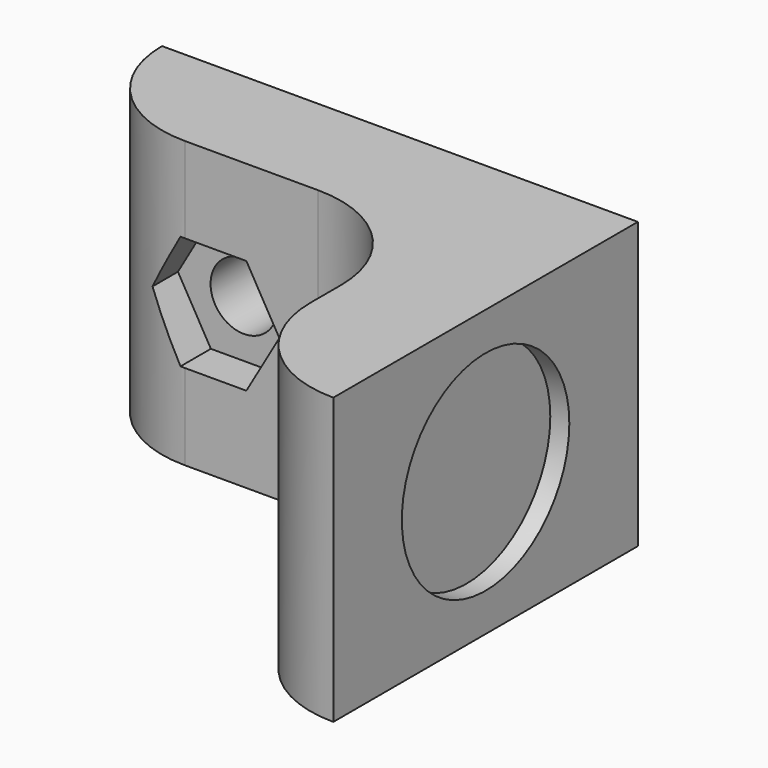
from build123d import *

# Parameters (mm, degrees)
F3_W         = 25
F3_H         = 15
F3_R         = 1.75
F4_DEPTH     = 6
F5_W         = 14
F5_H         = 15
F6_DEPTH     = 6
F7_R         = 5.5
F8_DEPTH     = 1
F9_R         = 1.75
F10_DEPTH    = 2
F11_T1_DEPTH = 15
F11_T3_DEPTH = 45


# Not quite as in the source:
# - a fillet or chamfer that OpenCascade refuses, or shapes differently, is made with other operations: its cross-section is extruded or revolved along the edge and cut away or added


with BuildPart() as f4:
    # F3 (on Front) → F4 (new body)
    with BuildSketch(Plane.XZ):
        with Locations((12.5, 7.5)):
            Rectangle(F3_W, F3_H)
        with Locations((7.5, 7.5)):
            Circle(F3_R, mode=Mode.SUBTRACT)
    extrude(amount=F4_DEPTH)

    # F5 (on face) → F6 (join)
    with BuildSketch(Plane.YZ.offset(25)):
        with Locations((-13, 7.5)):
            Rectangle(F5_W, F5_H)
    extrude(amount=-F6_DEPTH)

    # F7 (on face) → F8 (cut)
    with BuildSketch(Plane.YZ.offset(25)):
        with Locations((-10, 7.5)):
            Circle(F7_R)
    extrude(amount=-F8_DEPTH, mode=Mode.SUBTRACT)

    # F9 (on face) → F10 (cut)
    with BuildSketch(Plane.XZ.offset(6)):
        Polygon((10.9641016151, 7.5), (9.2320508076, 10.5), (5.7679491924, 10.5), (4.0358983849, 7.5), (5.7679491924, 4.5), (9.2320508076, 4.5), align=None)
        with Locations((7.5, 7.5)):
            Circle(F9_R, mode=Mode.SUBTRACT)
    extrude(amount=-F10_DEPTH, mode=Mode.SUBTRACT)

    # F11: fillet of radius 6 on 3 edges, made by hand

    # F11_s2 → F11_t1 (join)
    with BuildSketch(Plane.XY):
        with BuildLine():
            ThreePointArc((13, -6), (17.2426406871, -7.7573593129), (19, -12))
            Line((19, -12), (19, -6))
            Line((19, -6), (13, -6))
        make_face()
    extrude(amount=F11_T1_DEPTH)

    # F11_s4 → F11_t3 (cut)
    with BuildSketch(Plane.XY.offset(-15)):
        with BuildLine():
            ThreePointArc((0, 0), (1.7573593129, -4.2426406871), (6, -6))
            Line((6, -6), (0, -6))
            Line((0, -6), (0, 0))
        make_face()
        with BuildLine():
            ThreePointArc((25, -20), (20.7573593129, -18.2426406871), (19, -14))
            Line((19, -14), (19, -20))
            Line((19, -20), (25, -20))
        make_face()
    extrude(amount=F11_T3_DEPTH, mode=Mode.SUBTRACT)


solid = f4.part
